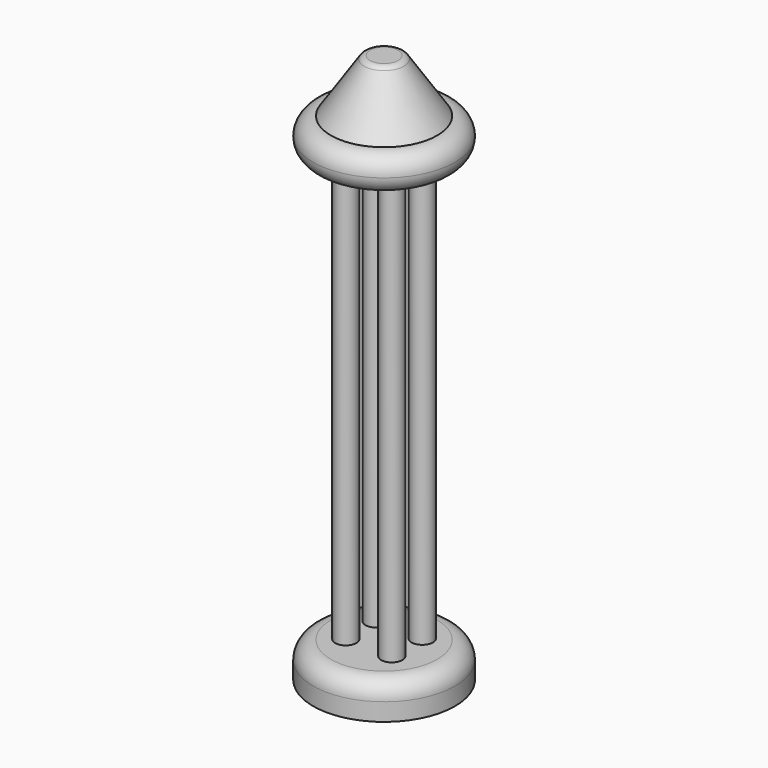
from build123d import *

# Parameters (mm, degrees)
F0_R      = 50.8
F1_DEPTH  = 25.4
F2_R      = 12.7
F3_R      = 7.62
F5_DEPTH  = 304.8
F4_R      = 7.62
F6_DEPTH  = 304.8
F8_R      = 50.8
F9_DEPTH  = 25.4
F10_R     = 12.7
F11_R     = 12.69999
F9_FACE_R = 38.10001
F22_R     = 12.7
F24_R     = 5.08


# Not quite as in the source:
# - a fillet or chamfer is up to 0.001 mm smaller than in the source, because OpenCascade refuses the exact size
# - the program builds the solid bodies; features that only make, move or delete a surface that nothing else refers to are left out


with BuildPart() as f1:
    # F0 (on Top) → F1 (new body)
    with BuildSketch(Plane.XY):
        Circle(F0_R)
    extrude(amount=F1_DEPTH)

    # F2
    f2_edges = [f1.edges().sort_by_distance(p)[0] for p in [
        (-50.8, 0, 25.4),
    ]]
    fillet(f2_edges, radius=F2_R)

    # F3 (on face) → F5 (join)
    with BuildSketch(Plane.XY.offset(25.4)):
        with Locations((-17.3765644431, 14.6533707157)):
            Circle(F3_R)
    extrude(amount=F5_DEPTH)

    # F4 (on face) → F6 (join)
    with BuildSketch(Plane.XY.offset(25.4)):
        with Locations((15.8204566687, 14.3940197304)):
            Circle(F4_R)
        with Locations((15.8195672557, -12.837909162)):
            Circle(F4_R)
        with Locations((-17.1172115952, -12.837909162)):
            Circle(F4_R)
    extrude(amount=F6_DEPTH)

    # F8 (on offset) → F9 (join)
    with BuildSketch(Plane.XY.offset(330.2)):
        Circle(F8_R)
    extrude(amount=F9_DEPTH)

    # F10
    f10_edges = [f1.edges().sort_by_distance(p)[0] for p in [
        (-50.8, 0, 330.2),
    ]]
    fillet(f10_edges, radius=F10_R)

    # F11 (radius 12.7 in the source; OpenCascade refuses exactly that, so slightly less here)
    f11_edges = [f1.edges().sort_by_distance(p)[0] for p in [
        (-50.8, 0, 355.6),
    ]]
    fillet(f11_edges, radius=F11_R)

    # F9_face (on face) → F23 section 0
    with BuildSketch(Plane.XY.offset(355.6)):
        Circle(F9_FACE_R)
    # F22 (on offset) → F23 section 1
    with BuildSketch(Plane.XY.offset(393.7)):
        Circle(F22_R)
    loft()

    # F24
    f24_edges = [f1.edges().sort_by_distance(p)[0] for p in [
        (-12.7, 0, 393.7),
    ]]
    fillet(f24_edges, radius=F24_R)


solid = f1.part
